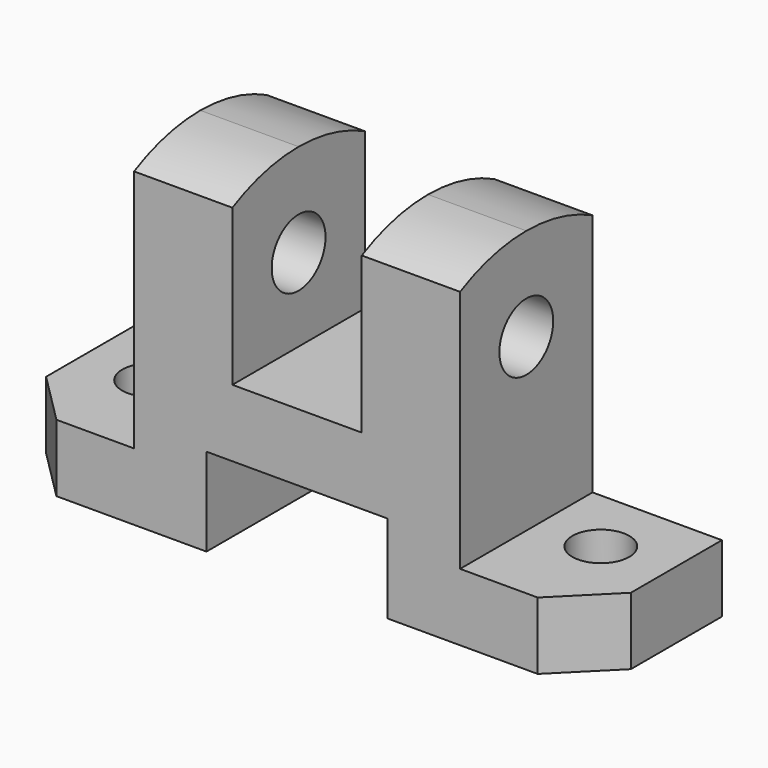
from build123d import *

# Parameters (mm, degrees)
F0_R     = 6.5
F1_DEPTH = 113
F2_W     = 25
F2_H     = 47.1287648325
F2_W_2   = 35
F2_H_2   = 17
F2_H_3   = 30.1287648325
F2_H_4   = 3.8712351675
F3_DEPTH = 32.001
F4_R     = 5.5
F5_DEPTH = 13.001
F6_SIZE  = 10


# Not quite as in the source:
# - a feature names something its author has since deleted; it is built from what else it names


with BuildPart() as f1:
    # F0 (on Right) → F1 (new body)
    with BuildSketch(Plane.YZ):
        with BuildLine():
            Line((0, 60.1287648325), (0, 0))
            Line((0, 0), (32, 0))
            Line((32, 0), (32, 60.1287648325))
            ThreePointArc((32, 60.1287648325), (24.2308332161, 63.0184271325), (16, 64))
            ThreePointArc((16, 64), (7.769166784, 63.0184271325), (0, 60.1287648325))
        make_face()
        with Locations((16, 46)):
            Circle(F0_R, mode=Mode.SUBTRACT)
    extrude(amount=F1_DEPTH)

    # F2 (on face) → F3 (cut, through all)
    with BuildSketch(Plane.XZ):
        with Locations((12.5, 36.5643824163)):
            Rectangle(F2_W, F2_H)
        with Locations((56.5, 8.5)):
            Rectangle(F2_W_2, F2_H_2)
        with Locations((100.5, 36.5643824163)):
            Rectangle(F2_W, F2_H)
        with Locations((56.5, 45.0643824163)):
            Rectangle(F2_W, F2_H_3)
        with Locations((12.5, 62.0643824163)):
            Rectangle(F2_W, F2_H_4)
        with Locations((56.5, 62.0643824163)):
            Rectangle(F2_W, F2_H_4)
        with Locations((100.5, 62.0643824163)):
            Rectangle(F2_W, F2_H_4)
    extrude(amount=-F3_DEPTH, mode=Mode.SUBTRACT)

    # F4 (on face) → F5 (cut, through all)
    with BuildSketch(Plane.XY.offset(13)):
        with Locations((100, 19)):
            Circle(F4_R)
        with Locations((13, 19)):
            Circle(F4_R)
    extrude(amount=-F5_DEPTH, mode=Mode.SUBTRACT)

    # F6
    f6_edges = [f1.edges().sort_by_distance(p)[0] for p in [
        (0, 0, 6.5),
        (113, 0, 6.5),
    ]]
    chamfer(f6_edges, length=F6_SIZE)


solid = f1.part
